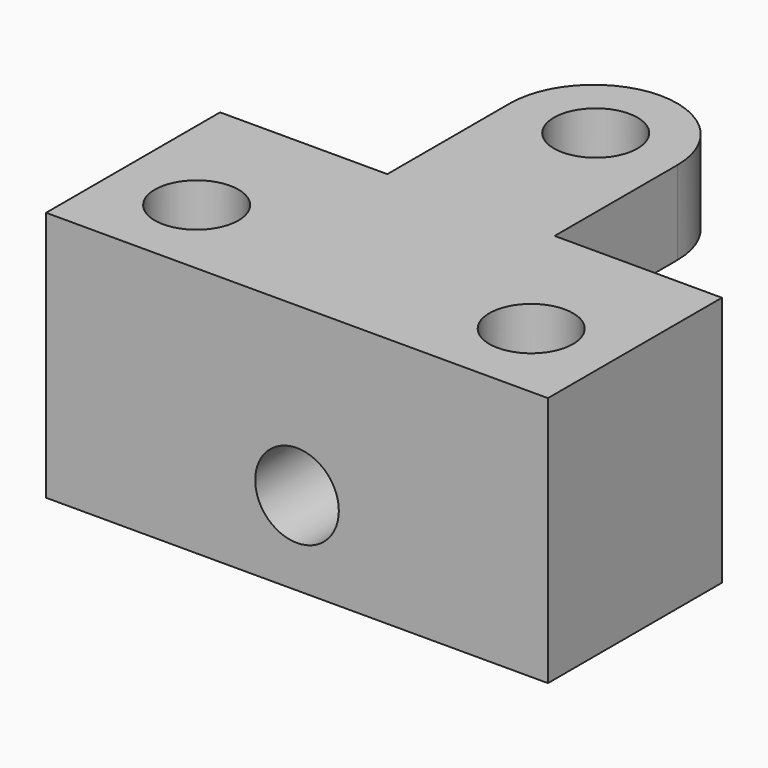
from build123d import *

# Parameters (mm, degrees)
F0_W      = 160
F0_H      = 160
F1_DEPTH  = 160
F4_W      = 300
F4_H      = 150
F5_DEPTH  = 130
F6_W      = 100
F6_H      = 143
F7_DEPTH  = 50
F8_R      = 25
F9_DEPTH  = 100
F10_R     = 25
F11_DEPTH = 50
F13_DEPTH = 50
F14_R     = 25
F15_DEPTH = 130


with BuildPart() as f1:
    # F0 (on Front) → F1 (new body)
    with BuildSketch(Plane.XZ):
        Rectangle(F0_W, F0_H)
    extrude(amount=F1_DEPTH)


with BuildPart() as f5:
    # F4 (on face) → F5 (new body)
    with BuildSketch(Plane(origin=(0, 0, 0), x_dir=(-1, 0, 0), z_dir=(0, 1, 0))):
        Rectangle(F4_W, F4_H)
    extrude(amount=F5_DEPTH)

    # F6 (on face) → F7 (join)
    with BuildSketch(Plane.XY.offset(75)):
        with Locations((0, 201.5)):
            Rectangle(F6_W, F6_H)
    extrude(amount=-F7_DEPTH)

    # F8 (on face) → F9 (cut)
    with BuildSketch(Plane.XY.offset(75)):
        with Locations((100, 50)):
            Circle(F8_R)
        with Locations((-100, 50)):
            Circle(F8_R)
    extrude(amount=-F9_DEPTH, mode=Mode.SUBTRACT)

    # F10 (on face) → F11 (cut)
    with BuildSketch(Plane.XY.offset(75)):
        with Locations((0, 223.2050807569)):
            Circle(F10_R)
    extrude(amount=-F11_DEPTH, mode=Mode.SUBTRACT)

    # F12 (on face) → F13 (cut)
    with BuildSketch(Plane.XY.offset(75)):
        with BuildLine():
            ThreePointArc((-50, 221.6448485851), (0, 271.6448485851), (50, 221.6448485851))
            Line((50, 221.6448485851), (50, 273))
            Line((50, 273), (-50, 273))
            Line((-50, 273), (-50, 221.6448485851))
        make_face()
    extrude(amount=-F13_DEPTH, mode=Mode.SUBTRACT)

    # F14 (on face) → F15 (cut)
    with BuildSketch(Plane.XZ):
        with Locations((0, -25)):
            Circle(F14_R)
    extrude(amount=-F15_DEPTH, mode=Mode.SUBTRACT)


solid = f5.part
